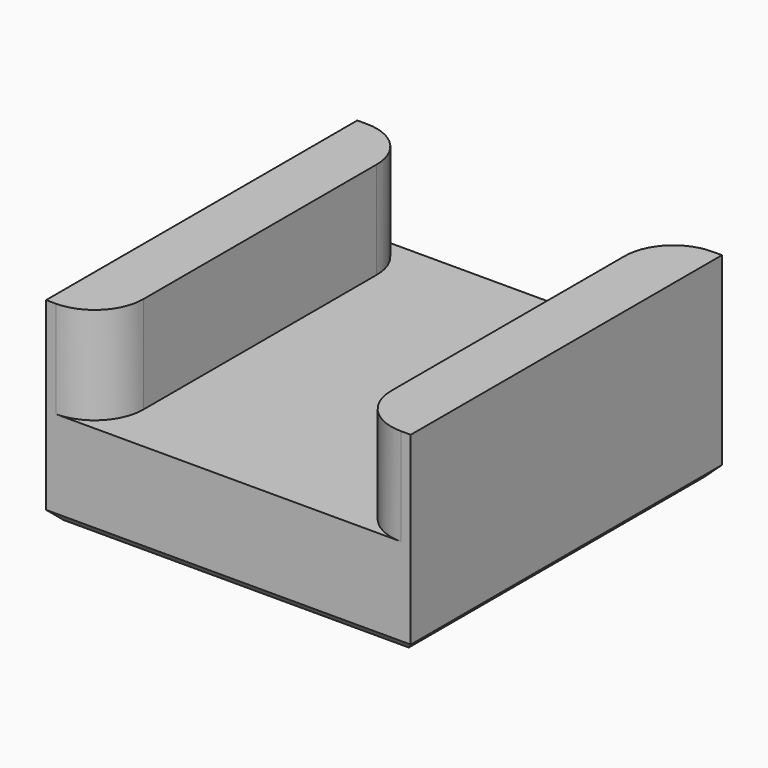
from build123d import *

# Parameters (mm, degrees)
F1_W    = 5.1
F1_H    = 8
F1_W_2  = 1.2
F4_R    = 1
F5_SIZE = 0.2


with BuildPart() as f2:
    # F2: sweep along a path in F0
    with BuildLine(Plane.XZ) as f2_path:
        Line((0, 0), (0, -2))
    # F1 (on Top) → F2 (sweep)
    with BuildSketch(Plane.XY):
        Rectangle(F1_W, F1_H)
        with Locations((3.15, 0)):
            Rectangle(F1_W_2, F1_H)
        with Locations((-3.15, 0)):
            Rectangle(F1_W_2, F1_H)
    sweep(path=f2_path.line)

    # F3: sweep along a path in F0
    with BuildLine(Plane.XZ) as f3_path:
        Line((0, 0), (0, 1.9990060536))
    # F1 (on Top) → F3 (sweep)
    with BuildSketch(Plane.XY):
        with Locations((-3.15, 0)):
            Rectangle(F1_W_2, F1_H)
        with Locations((3.15, 0)):
            Rectangle(F1_W_2, F1_H)
    sweep(path=f3_path.line)

    # F4
    f4_edges = [f2.edges().sort_by_distance(p)[0] for p in [
        (-2.55, 4, 0.999503),
        (2.55, 4, 0.999503),
        (2.55, -4, 0.999503),
        (-2.55, -4, 0.999503),
    ]]
    fillet(f4_edges, radius=F4_R)

    # F5
    f5_edges = [f2.edges().sort_by_distance(p)[0] for p in [
        (0, -4, -2),
        (3.75, 0, -2),
        (0, 4, -2),
        (-3.75, 0, -2),
    ]]
    chamfer(f5_edges, length=F5_SIZE)


solid = f2.part
